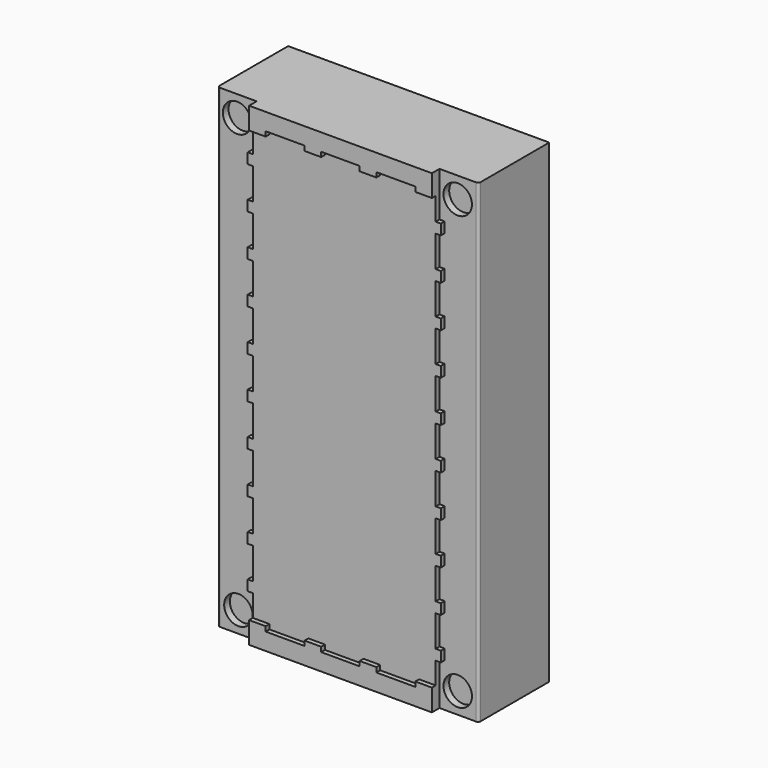
from build123d import *

# Parameters (mm, degrees)
F0_W      = 27.5
F0_H      = 50
F1_DEPTH  = 9.3
F3_DEPTH  = 0.5
F4_R      = 1.5
F5_DEPTH  = 0.75
F6_R      = 0.25
F8_DEPTH  = 0.5
F9_W      = 17.5
F9_H      = 40
F10_DEPTH = 5
F11_SIZE  = 0.5


with BuildPart() as f1:
    # F0 (on Front) → F1 (new body)
    with BuildSketch(Plane.XZ):
        with Locations((13.75, 25)):
            Rectangle(F0_W, F0_H)
    extrude(amount=F1_DEPTH)

    # F2 (on face) → F3 (join)
    with BuildSketch(Plane.XZ.offset(9.3)):
        Polygon((13.75, 50), (4.1195944277, 50), (4.1195944277, 45.3), (3.5795944277, 45.3), (3.5795944277, 44.2), (4.1195944277, 44.2), (4.1195944277, 40.9), (3.5795944277, 40.9), (3.5795944277, 39.8), (4.1195944277, 39.8), (4.1195944277, 36.5), (3.5795944277, 36.5), (3.5795944277, 35.4), (4.1195944277, 35.4), (4.1195944277, 32.1), (3.5795944277, 32.1), (3.5795944277, 31), (4.1195944277, 31), (4.1195944277, 27.7), (3.5795944277, 27.7), (3.5795944277, 26.6), (4.1195944277, 26.6), (4.1195944277, 23.3), (3.5795944277, 23.3), (3.5795944277, 22.2), (4.1195944277, 22.2), (4.1195944277, 18.9), (3.5795944277, 18.9), (3.5795944277, 17.8), (4.1195944277, 17.8), (4.1195944277, 14.5), (3.5795944277, 14.5), (3.5795944277, 13.4), (4.1195944277, 13.4), (4.1195944277, 10.1), (3.5795944277, 10.1), (3.5795944277, 9), (4.1195944277, 9), (4.1195944277, 5.7), (3.5795944277, 5.7), (3.5795944277, 4.6), (4.1195944277, 4.6), (4.1195944277, 0), (13.75, 0), (23.3804055723, 0), (23.3804055723, 4.6), (23.9204055723, 4.6), (23.9204055723, 5.7), (23.3804055723, 5.7), (23.3804055723, 9), (23.9204055723, 9), (23.9204055723, 10.1), (23.3804055723, 10.1), (23.3804055723, 13.4), (23.9204055723, 13.4), (23.9204055723, 14.5), (23.3804055723, 14.5), (23.3804055723, 17.8), (23.9204055723, 17.8), (23.9204055723, 18.9), (23.3804055723, 18.9), (23.3804055723, 22.2), (23.9204055723, 22.2), (23.9204055723, 23.3), (23.3804055723, 23.3), (23.3804055723, 26.6), (23.9204055723, 26.6), (23.9204055723, 27.7), (23.3804055723, 27.7), (23.3804055723, 31), (23.9204055723, 31), (23.9204055723, 32.1), (23.3804055723, 32.1), (23.3804055723, 35.4), (23.9204055723, 35.4), (23.9204055723, 36.5), (23.3804055723, 36.5), (23.3804055723, 39.8), (23.9204055723, 39.8), (23.9204055723, 40.9), (23.3804055723, 40.9), (23.3804055723, 44.2), (23.9204055723, 44.2), (23.9204055723, 45.3), (23.3804055723, 45.3), (23.3804055723, 50), align=None)
    extrude(amount=F3_DEPTH)

    # F4 (on face) → F5 (cut)
    with BuildSketch(Plane.XZ.offset(9.3)):
        with Locations((2.2, 2.2)):
            Circle(F4_R)
        with Locations((25.3, 2.2)):
            Circle(F4_R)
        with Locations((2.0597972139, 47.8)):
            Circle(F4_R)
        with Locations((25.3, 47.8)):
            Circle(F4_R)
    extrude(amount=-F5_DEPTH, mode=Mode.SUBTRACT)

    # F6
    f6_edges = [f1.edges().sort_by_distance(p)[0] for p in [
        (0, -9.3, 25),
        (27.5, -9.3, 25),
    ]]
    fillet(f6_edges, radius=F6_R)

    # F7 (on face) → F8 (join)
    with BuildSketch(Plane.XZ.offset(9.8)):
        Polygon((23.3804055723, 50), (4.1195944277, 50), (4.1195944277, 48.2), (4.1195944277, 47.7), (5.8695944277, 47.7), (5.8695944277, 48.2), (9.9695944277, 48.2), (9.9695944277, 47.7), (11.7195944277, 47.7), (11.7195944277, 48.2), (15.7804055723, 48.2), (15.7804055723, 47.7), (17.5304055723, 47.7), (17.5304055723, 48.2), (21.6304055723, 48.2), (21.6304055723, 47.7), (23.3804055723, 47.7), (23.3804055723, 48.2), align=None)
        Polygon((23.3804055723, 2.3), (21.6304055723, 2.3), (21.6304055723, 1.8), (17.5304055723, 1.8), (17.5304055723, 2.3), (15.7804055723, 2.3), (15.7804055723, 1.8), (11.7195944277, 1.8), (11.7195944277, 2.3), (9.9695944277, 2.3), (9.9695944277, 1.8), (5.8695944277, 1.8), (5.8695944277, 2.3), (4.1195944277, 2.3), (4.1195944277, 1.8), (4.1195944277, 0), (23.3804055723, 0), (23.3804055723, 1.8), align=None)
    extrude(amount=F8_DEPTH)

    # F9 (on face) → F10 (cut)
    with BuildSketch(Plane.XZ):
        with Locations((13.75, 25)):
            Rectangle(F9_W, F9_H)
    extrude(amount=F10_DEPTH, mode=Mode.SUBTRACT)

    # F11
    f11_edges = [f1.edges().sort_by_distance(p)[0] for p in [
        (5, -2.5, 45),
        (13.75, -5, 45),
        (5, -5, 25),
        (22.5, -5, 25),
        (5, -2.5, 5),
        (13.75, -5, 5),
        (22.5, -2.5, 5),
        (13.75, 0, 5),
        (22.5, -2.5, 45),
        (13.75, 0, 45),
        (5, 0, 25),
        (22.5, 0, 25),
    ]]
    chamfer(f11_edges, length=F11_SIZE)


solid = f1.part
